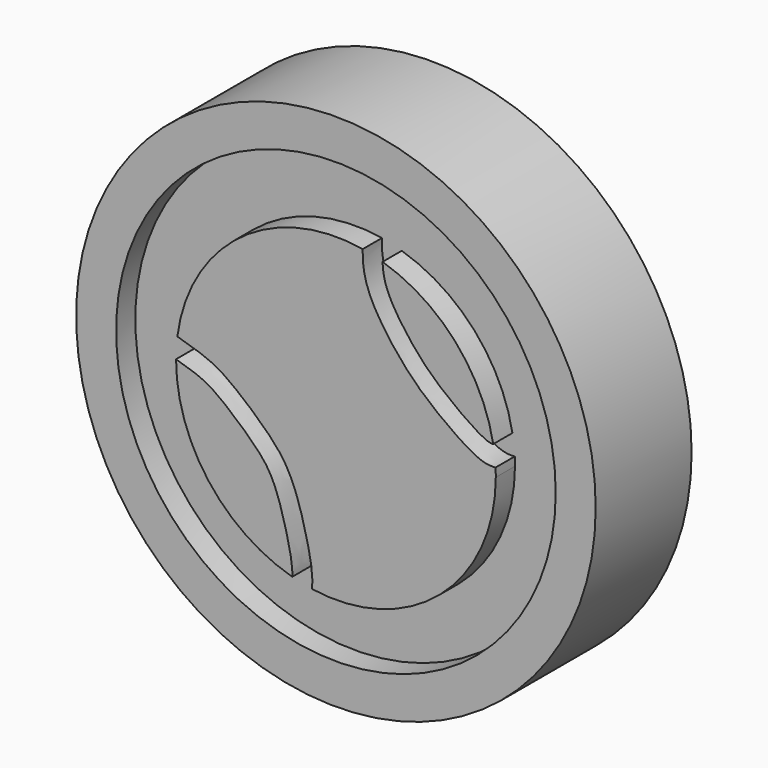
from build123d import *

# Parameters (mm, degrees)
F1_R     = 6.5
F1_R_2   = 5.5
F3_DEPTH = 3
F4_DEPTH = 1.5
F5_DEPTH = 0.6
F6_DEPTH = 1
F7_DEPTH = 1
F8_DEPTH = 1


# Not quite as in the source:
# - ends of sketch curves that miss each other by under 0.0002 mm in the source are joined
# - the dataset's text gives a spline's control points without its knots; the knots are read off the source's solid


with BuildPart() as f3:
    # F1 (on Front) → F3 (new body)
    with BuildSketch(Plane.XZ):
        with Locations((1.996e-07, 0.145563783)):
            Circle(F1_R)
        with Locations((1.996e-07, 0.145563783)):
            Circle(F1_R_2, mode=Mode.SUBTRACT)
    extrude(amount=-F3_DEPTH)

    # F0 (on Front) + F1 (on Front) → F4 (join)
    with BuildSketch(Plane.XZ):
        with BuildLine():
            add(Edge.make_bspline(
                [(-1.4633628161, -3.8408698747), (-0.8618942381, -4.0797628795), (1.7775925035, -4.2725148883), (2.1266039699, -2.4883414841), (2.1792066492, -0.8570773415), (2.1261946367, 0.7652860278), (1.8591945487, 1.4152828688), (2.1073079889, 1.4090746613), (2.1070261206, 1.5973545621), (1.8482611221, 1.6571502022), (1.9106924097, 2.0013449435), (1.883292753, 2.4559971082), (1.4530608962, 2.5796008165), (1.3486705812, 2.982608362), (0.9522813685, 3.1051443516), (0.6376593936, 3.1670181532), (0.4331394013, 3.4063180529), (0.6426984155, 3.8176132891), (0.3981993423, 4.2634916825), (-0.0062082347, 4.3047771669), (-0.3006353253, 4.2313929361), (-0.6271454426, 3.9609581822), (-0.5601436399, 3.6082200906), (-0.4158755178, 3.3585569408), (-0.6804152796, 3.1141950016), (-1.0068060059, 3.1249120402), (-1.1963426018, 2.8920399235), (-1.3913162215, 2.8683333491), (-1.3804892819, 2.6236576239), (-1.7077578499, 2.7520009173), (-1.8276300328, 2.3206081403), (-1.8540486856, 2.0110635487), (-1.8641412125, 1.6986764558), (-2.1169141262, 1.6232767981), (-2.0818952059, 1.4062115725), (-1.9001690611, 1.4703026422), (-2.1146422172, 0.8809803752), (-2.0979861646, 0.2234423606), (-2.2011740498, -0.523800053), (-2.1724225003, -1.2230030424), (-2.1779022447, -2.5473945892), (-1.9120269544, -3.4285716282), (-1.7403824301, -3.7308424346), (-1.4633628161, -3.8408698747)],
                knots=[0, 0, 0, 0, 0.0614284178, 0.105210304, 0.1528188952, 0.1998934744, 0.2260159491, 0.2394622475, 0.2521789794, 0.2685961982, 0.2887254165, 0.3121716538, 0.3345624104, 0.3566054098, 0.3791085644, 0.3997521347, 0.4178904262, 0.4412373911, 0.4652934844, 0.487296569, 0.5074239254, 0.5296841222, 0.5504706917, 0.5687295132, 0.5882529988, 0.6087082105, 0.6278548545, 0.642595893, 0.6569229468, 0.674176944, 0.6961346625, 0.7176137944, 0.736576695, 0.7535032789, 0.767308469, 0.7778501968, 0.8029343179, 0.8341377518, 0.8649078271, 0.8956216456, 0.9374997946, 0.9717077879, 1, 1, 1, 1], degree=3))
        make_face()
    with BuildSketch(Plane.XZ):
        with Locations((1.996e-07, 0.145563783)):
            Circle(F1_R_2)
    extrude(amount=-F4_DEPTH)

    # F1 (on Front) + F0 (on Front) → F5 (cut)
    with BuildSketch(Plane.XZ):
        with Locations((1.996e-07, 0.145563783)):
            Circle(F1_R_2)
    with BuildSketch(Plane.XZ):
        with BuildLine():
            add(Edge.make_bspline(
                [(-1.4633628161, -3.8408698747), (-0.8618942381, -4.0797628795), (1.7775925035, -4.2725148883), (2.1266039699, -2.4883414841), (2.1792066492, -0.8570773415), (2.1261946367, 0.7652860278), (1.8591945487, 1.4152828688), (2.1073079889, 1.4090746613), (2.1070261206, 1.5973545621), (1.8482611221, 1.6571502022), (1.9106924097, 2.0013449435), (1.883292753, 2.4559971082), (1.4530608962, 2.5796008165), (1.3486705812, 2.982608362), (0.9522813685, 3.1051443516), (0.6376593936, 3.1670181532), (0.4331394013, 3.4063180529), (0.6426984155, 3.8176132891), (0.3981993423, 4.2634916825), (-0.0062082347, 4.3047771669), (-0.3006353253, 4.2313929361), (-0.6271454426, 3.9609581822), (-0.5601436399, 3.6082200906), (-0.4158755178, 3.3585569408), (-0.6804152796, 3.1141950016), (-1.0068060059, 3.1249120402), (-1.1963426018, 2.8920399235), (-1.3913162215, 2.8683333491), (-1.3804892819, 2.6236576239), (-1.7077578499, 2.7520009173), (-1.8276300328, 2.3206081403), (-1.8540486856, 2.0110635487), (-1.8641412125, 1.6986764558), (-2.1169141262, 1.6232767981), (-2.0818952059, 1.4062115725), (-1.9001690611, 1.4703026422), (-2.1146422172, 0.8809803752), (-2.0979861646, 0.2234423606), (-2.2011740498, -0.523800053), (-2.1724225003, -1.2230030424), (-2.1779022447, -2.5473945892), (-1.9120269544, -3.4285716282), (-1.7403824301, -3.7308424346), (-1.4633628161, -3.8408698747)],
                knots=[0, 0, 0, 0, 0.0614284178, 0.105210304, 0.1528188952, 0.1998934744, 0.2260159491, 0.2394622475, 0.2521789794, 0.2685961982, 0.2887254165, 0.3121716538, 0.3345624104, 0.3566054098, 0.3791085644, 0.3997521347, 0.4178904262, 0.4412373911, 0.4652934844, 0.487296569, 0.5074239254, 0.5296841222, 0.5504706917, 0.5687295132, 0.5882529988, 0.6087082105, 0.6278548545, 0.642595893, 0.6569229468, 0.674176944, 0.6961346625, 0.7176137944, 0.736576695, 0.7535032789, 0.767308469, 0.7778501968, 0.8029343179, 0.8341377518, 0.8649078271, 0.8956216456, 0.9374997946, 0.9717077879, 1, 1, 1, 1], degree=3))
        make_face()
    extrude(amount=-F5_DEPTH, mode=Mode.SUBTRACT)

    # F2 (on face) → F6 (join)
    with BuildSketch(Plane.XZ):
        with BuildLine():
            ThreePointArc((-0.6012813019, -3.9545493796), (2.6071895589, -3.0335725809), (4, 0))
            ThreePointArc((4, 0), (3.9985637458, 0.1071819529), (3.9942560145, 0.2142869356))
            add(Edge.make_bspline(
                [(0.6696937898, 3.9435403165), (0.6582621326, 3.6561648877), (0.748660393, 2.9819733395), (1.5906344476, 1.8060597163), (2.343729672, 1.0651587443), (3.5468225291, 0.2060757034), (3.8886131662, 0.2055288721), (3.9942560145, 0.2142869356)],
                knots=[0, 0, 0, 0, 0.1914441273, 0.4252731611, 0.6392341909, 0.8752207587, 1, 1, 1, 1], degree=3))
            ThreePointArc((0.6696937898, 3.9435403165), (-2.3798948862, 3.2149806112), (-3.9672180841, 0.5110583855))
            add(Edge.make_bspline(
                [(-3.9672180841, 0.5110583855), (-3.2570424953, 0.3072051337), (-2.8281277347, 0.1183736874), (-1.7521563519, -0.7910134795), (-1.1021707585, -1.5327189765), (-0.7270922455, -2.8181587186), (-0.5608016797, -3.6356710711), (-0.6012813019, -3.9545493796)],
                knots=[0, 0, 0, 0, 0.2105751714, 0.4131601255, 0.5959388752, 0.8062823722, 1, 1, 1, 1], degree=3))
        make_face()
    extrude(amount=-F6_DEPTH)

    # F2 (on face) → F7 (join)
    with BuildSketch(Plane.XZ):
        with BuildLine():
            ThreePointArc((-4, -5.4666e-06), (-3.1915709466, -2.4111978128), (-1.0930678122, -3.8477529492))
            add(Edge.make_bspline(
                [(-4, -5.4666e-06), (-3.8428166733, -0.0460123585), (-3.5603914777, -0.133738653), (-3.2985794295, -0.2386569495), (-3.1472677408, -0.3246867621), (-2.9956539452, -0.4287257802), (-2.8222463482, -0.557104318), (-2.5840878529, -0.7485534177), (-2.2954985412, -1.0016010876), (-2.036026908, -1.2482860637), (-1.8381629968, -1.4634144564), (-1.6835113586, -1.6757370022), (-1.5516009911, -1.9240469669), (-1.4256566149, -2.248184411), (-1.3146225307, -2.6109466281), (-1.2146554645, -2.9978949757), (-1.1313238625, -3.3629451013), (-1.0901758206, -3.651388342), (-1.0894246902, -3.7951254649), (-1.0930678122, -3.8477529492)],
                knots=[0.0110273175, 0.0110273175, 0.0110273175, 0.0110273175, 0.0625, 0.125, 0.1875, 0.21875, 0.25, 0.3125, 0.375, 0.4375, 0.5, 0.5625, 0.625, 0.6875, 0.75, 0.8125, 0.875, 0.9375, 0.9857876166, 0.9857876166, 0.9857876166, 0.9857876166], degree=3))
        make_face()
    extrude(amount=-F7_DEPTH)

    # F2 (on face) → F8 (join)
    with BuildSketch(Plane.XZ):
        with BuildLine():
            add(Edge.make_bspline(
                [(1.1680500995, 3.8256503793), (1.1697995693, 3.7107206965), (1.1918189199, 3.5214057887), (1.2802032379, 3.2411969251), (1.4118748463, 2.9720045965), (1.5937127908, 2.679461535), (1.8023614597, 2.3919954972), (2.0179930746, 2.1262894096), (2.2181018419, 1.9032227167), (2.4259640622, 1.6986298437), (2.6643415193, 1.4905337309), (2.9597106264, 1.2554890784), (3.2786287368, 1.0236228812), (3.5292013722, 0.8637020638), (3.6951311872, 0.7741756792), (3.7886457426, 0.7328710188), (3.8426743367, 0.7168415355), (3.8851876888, 0.7098421735), (3.9097876849, 0.7094994811), (3.9362444503, 0.7113026549)],
                knots=[0.0276671484, 0.0276671484, 0.0276671484, 0.0276671484, 0.125, 0.1875, 0.25, 0.3125, 0.375, 0.4375, 0.5, 0.5625, 0.625, 0.6875, 0.75, 0.8125, 0.84375, 0.875, 0.90625, 0.9375, 0.9898649034, 0.9898649034, 0.9898649034, 0.9898649034], degree=3))
            ThreePointArc((3.9362444503, 0.7113026549), (2.989694007, 2.6573915302), (1.1680500995, 3.8256503793))
        make_face()
    extrude(amount=-F8_DEPTH)


solid = f3.part
